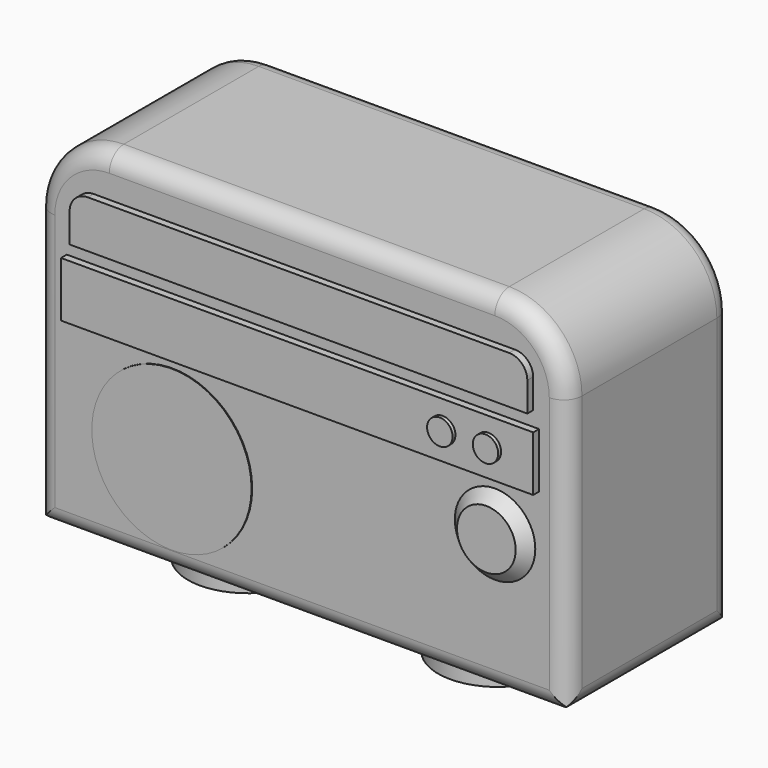
from build123d import *

# Parameters (mm, degrees)
F1_DEPTH     = 56.4
F4_W         = 129.9849450588
F4_H         = 15.1807228103
F5_DEPTH     = 2
F6_R         = 3.5
F7_DEPTH     = 1
F2_R         = 16.4693442444
F8_DEPTH     = 8
F3_R         = 13.0758852418
F9_DEPTH     = 3
F11_DEPTH    = 2
F34_R        = 5
F35_R        = 5
F36_T1_DEPTH = 71.4
F37_T1_DEPTH = 71.4
F40_R        = 21.9971090936
F41_DEPTH    = 0.2


# Not quite as in the source:
# - a fillet or chamfer that OpenCascade refuses, or shapes differently, is made with other operations: its cross-section is extruded or revolved along the edge and cut away or added
# - the program builds the solid bodies; features that only make, move or delete a surface that nothing else refers to are left out


with BuildPart() as f1:
    # F0 (on Front) → F1 (new body)
    with BuildSketch(Plane.XZ):
        with BuildLine():
            Line((52.9453340173, 52.3588129878), (-53.1794461608, 52.3588129878))
            ThreePointArc((-53.1794461608, 52.3588129878), (-67.3215817845, 46.5009486115), (-73.1794461608, 32.3588129878))
            Line((-73.1794461608, 32.3588129878), (-73.1794461608, -43.5259789228))
            Line((-73.1794461608, -43.5259789228), (72.9453340173, -43.5259789228))
            Line((72.9453340173, -43.5259789228), (72.9453340173, 32.3588129878))
            ThreePointArc((72.9453340173, 32.3588129878), (67.087469641, 46.5009486115), (52.9453340173, 52.3588129878))
        make_face()
    extrude(amount=-F1_DEPTH)

    # F34
    f34_edges = [f1.edges().sort_by_distance(p)[0] for p in [
        (-0.117056, 0, 52.358813),
        (-67.321582, 0, 46.500949),
        (-73.179446, 0, -5.583583),
        (-0.117056, 0, -43.525979),
        (72.945334, 0, -5.583583),
        (67.08747, 0, 46.500949),
    ]]
    fillet(f34_edges, radius=F34_R)

    # F35
    f35_edges = [f1.edges().sort_by_distance(p)[0] for p in [
        (-0.117056, 56.4, 52.358813),
        (-67.321582, 56.4, 46.500949),
        (-73.179446, 56.4, -5.583583),
        (-0.117056, 56.4, -43.525979),
        (72.945334, 56.4, -5.583583),
        (67.08747, 56.4, 46.500949),
    ]]
    fillet(f35_edges, radius=F35_R)

    # F36: fillet of radius 5 on 4 edges, made by hand

    # F36_s2 → F36_t1 (cut)
    with BuildSketch(Plane.XZ.offset(-63.9)):
        with BuildLine():
            ThreePointArc((72.9453340173, -38.5259789228), (71.4808679232, -42.0615128288), (67.9453340173, -43.5259789228))
            Line((67.9453340173, -43.5259789228), (72.9453340173, -43.5259789228))
            Line((72.9453340173, -43.5259789228), (72.9453340173, -38.5259789228))
        make_face()
    extrude(amount=F36_T1_DEPTH, mode=Mode.SUBTRACT)

    # F37: fillet of radius 5 on 4 edges, made by hand

    # F37_s2 → F37_t1 (cut)
    with BuildSketch(Plane.XZ.offset(-63.9)):
        with BuildLine():
            ThreePointArc((-73.1794461608, -38.5259789228), (-71.7149800667, -42.0615128288), (-68.1794461608, -43.5259789228))
            Line((-68.1794461608, -43.5259789228), (-73.1794461608, -43.5259789228))
            Line((-73.1794461608, -43.5259789228), (-73.1794461608, -38.5259789228))
        make_face()
    extrude(amount=F37_T1_DEPTH, mode=Mode.SUBTRACT)


with BuildPart() as f5:
    # F4 (on face) → F5 (new body)
    with BuildSketch(Plane.XZ):
        with Locations((0.1185983419, 16.2481176667)):
            Rectangle(F4_W, F4_H)
    extrude(amount=F5_DEPTH)


with BuildPart() as f7:
    # F6 (on face) → F7 (new body)
    with BuildSketch(Plane.XZ.offset(2)):
        with Locations((52.7767315507, 16.2481181324)):
            Circle(F6_R)
    extrude(amount=F7_DEPTH)


with BuildPart() as f7b:
    # F6 (on face) → F7, piece 2 (new body)
    with BuildSketch(Plane.XZ.offset(2)):
        with Locations((40.2051955462, 16.2481181324)):
            Circle(F6_R)
    extrude(amount=F7_DEPTH)


with BuildPart() as f8:
    # F2 (on face) → F8 (new body)
    with BuildSketch(Plane(origin=(0, 0, -43.5259789228), x_dir=(1, 0, 0), z_dir=(0, 0, -1))):
        with Locations((-36.7238521576, -27.0820427686)):
            Circle(F2_R)
    extrude(amount=F8_DEPTH)


with BuildPart() as f8b:
    # F2 (on face) → F8, piece 2 (new body)
    with BuildSketch(Plane(origin=(0, 0, -43.5259789228), x_dir=(1, 0, 0), z_dir=(0, 0, -1))):
        with Locations((32.5050577521, -26.614209637)):
            Circle(F2_R)
    extrude(amount=F8_DEPTH)


with BuildPart() as f9:
    # F3 (on face) → F9 (new body)
    with BuildSketch(Plane.XZ):
        with Locations((53.0139356852, -5.5835829675)):
            Circle(F3_R)
    extrude(amount=F9_DEPTH)

    # F29: chamfer of 5 on 1 edges, made by hand

    # F29_s1 → F29_t2 (revolve, cut)
    with BuildSketch(Plane.XY.offset(-5.5835829675)):
        Polygon((66.089820927, 2), (61.089820927, -3), (66.089820927, -3), align=None)
    revolve(axis=Axis((53.0139356852, -3, -5.5835829675), (0, -1, 0)), mode=Mode.SUBTRACT)


with BuildPart() as f11:
    # F10 (on face) → F11 (new body)
    with BuildSketch(Plane.XZ):
        with BuildLine():
            Line((58.4981150031, 40.9356179833), (-57.5018849969, 40.9356179833))
            ThreePointArc((-57.5018849969, 40.9356179833), (-61.0374189028, 39.4711518893), (-62.5018849969, 35.9356179833))
            Line((-62.5018849969, 35.9356179833), (-62.5018849969, 27.8708599508))
            Line((-62.5018849969, 27.8708599508), (63.4981150031, 27.8708599508))
            Line((63.4981150031, 27.8708599508), (63.4981150031, 35.9356179833))
            ThreePointArc((63.4981150031, 35.9356179833), (62.033648909, 39.4711518893), (58.4981150031, 40.9356179833))
        make_face()
    extrude(amount=F11_DEPTH)


with BuildPart() as f41:
    # F40 (on face) → F41 (new body)
    with BuildSketch(Plane.XZ):
        with Locations((-35.8415655792, -16.2585619837)):
            Circle(F40_R)
    extrude(amount=F41_DEPTH)


solid = Compound([f1.part, f5.part, f7.part, f7b.part, f8.part, f8b.part, f9.part, f11.part, f41.part])
